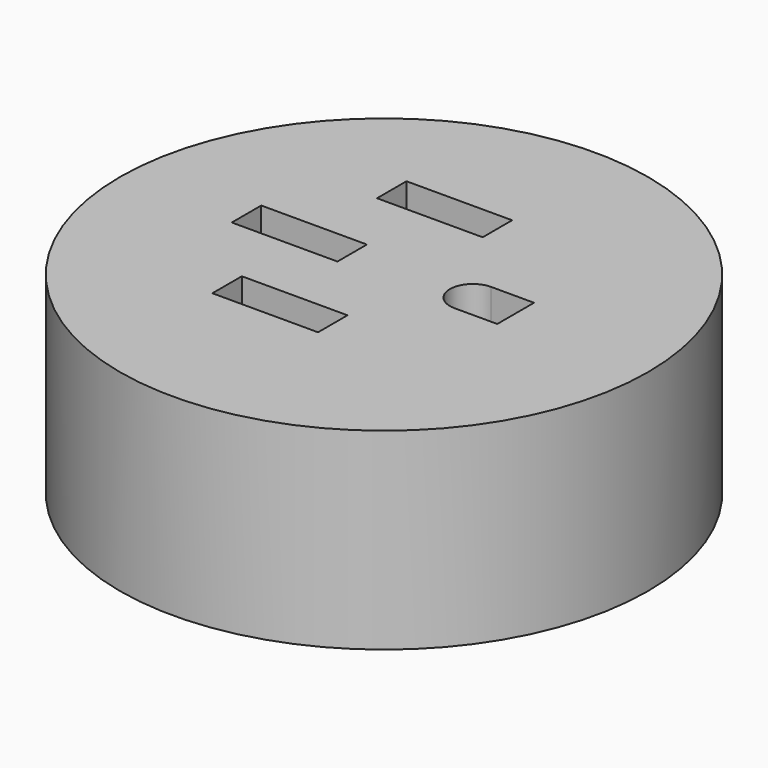
from build123d import *

# Parameters (mm, degrees)
F0_R     = 24.66759
F0_W     = 9.8689098377
F0_H     = 3.4395875409
F0_W_2   = 9.86891
F0_H_2   = 3.43959
F1_DEPTH = 18.8
F2_DEPTH = 0.8


# Not quite as in the source:
# - a feature names something its author has since deleted; it is built from what else it names


with BuildPart() as f1:
    # F0 (on Top) → F1 (new body)
    with BuildSketch(Plane.XY):
        Circle(F0_R)
        with Locations((-2.9931267491, -8.4071261808)):
            Rectangle(F0_W, F0_H, mode=Mode.SUBTRACT)
        with Locations((-8.8684857703, 1.2023462914)):
            Rectangle(F0_W_2, F0_H_2, mode=Mode.SUBTRACT)
        with Locations((-2.9931267491, 10.8118187636)):
            Rectangle(F0_W, F0_H, mode=Mode.SUBTRACT)
        with BuildLine():
            Line((11.3292662427, 3.3551587258), (11.3292662427, -0.9376045782))
            Line((11.3292662427, -0.9376045782), (7.332555484, -0.9376045782))
            ThreePointArc((7.332555484, -0.9376045782), (5.186173832, 1.2087770738), (7.332555484, 3.3551587258))
            Line((7.332555484, 3.3551587258), (11.3292662427, 3.3551587258))
        make_face(mode=Mode.SUBTRACT)
    extrude(amount=F1_DEPTH)

    # F0 (on Top) → F2 (cut)
    with BuildSketch(Plane.XY):
        Circle(F0_R)
        with Locations((-2.9931267491, -8.4071261808)):
            Rectangle(F0_W, F0_H, mode=Mode.SUBTRACT)
        with Locations((-8.8684857703, 1.2023462914)):
            Rectangle(F0_W_2, F0_H_2, mode=Mode.SUBTRACT)
        with Locations((-2.9931267491, 10.8118187636)):
            Rectangle(F0_W, F0_H, mode=Mode.SUBTRACT)
        with BuildLine():
            Line((11.3292662427, 3.3551587258), (11.3292662427, -0.9376045782))
            Line((11.3292662427, -0.9376045782), (7.332555484, -0.9376045782))
            ThreePointArc((7.332555484, -0.9376045782), (5.186173832, 1.2087770738), (7.332555484, 3.3551587258))
            Line((7.332555484, 3.3551587258), (11.3292662427, 3.3551587258))
        make_face(mode=Mode.SUBTRACT)
        with Locations((-2.9931267491, -8.4071261808)):
            Rectangle(F0_W, F0_H)
    extrude(amount=F2_DEPTH, mode=Mode.SUBTRACT)


solid = f1.part
